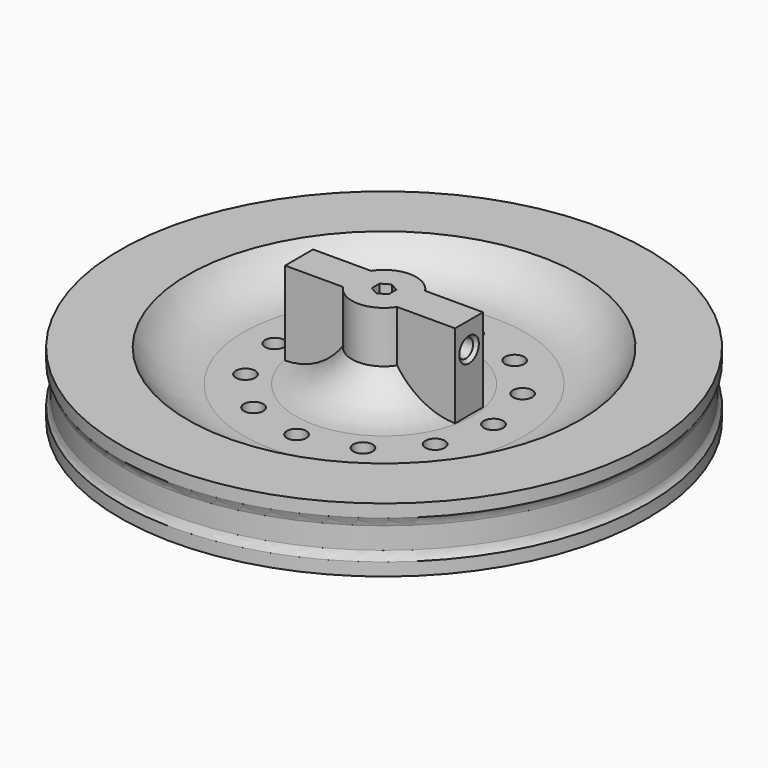
from build123d import *

# Parameters (mm, degrees)
F5_DEPTH  = 8
F6_DEPTH  = 9
F7_R      = 1.4
F8_DEPTH  = 54.201
F10_DEPTH = 18.001
F12_DEPTH = 26.4
F14_DEPTH = 18.001
F16_DEPTH = 5
F17_SIZE  = 0.5
F18_R     = 1.5
F19_DEPTH = 18.0010001


# Not quite as in the source:
# - a fillet or chamfer that OpenCascade refuses, or shapes differently, is made with other operations: its cross-section is extruded or revolved along the edge and cut away or added


with BuildPart() as f1:
    # F0 (on Front) → F1 (revolve)
    with BuildSketch(Plane.XZ):
        Polygon((0, 10), (0, 0), (41, 0), (41, 2), (40.5, 2), (40.5, 8), (41, 8), (41, 10), (30.5, 10), (30.5, 5), (5, 5), (5, 10), align=None)
    revolve(axis=Axis((0, 0, 5), (0, 0, -1)))

    # F2: fillet of radius 10 on 1 edges, made by hand

    # F2_s1 → F2_t2 (revolve)
    with BuildSketch(Plane.XZ):
        with BuildLine():
            ThreePointArc((13.6602540378, 5), (8.6602540378, 6.3397459622), (5, 10))
            Line((5, 10), (5, 5))
            Line((5, 5), (13.6602540378, 5))
        make_face()
    revolve(axis=Axis((0, 0, 5), (0, 0, -1)))

    # F3: fillet of radius 10 on 1 edges, made by hand

    # F3_s1 → F3_t2 (revolve)
    with BuildSketch(Plane.XZ):
        with BuildLine():
            ThreePointArc((30.5, 10), (26.8397459622, 6.3397459622), (21.8397459622, 5))
            Line((21.8397459622, 5), (30.5, 5))
            Line((30.5, 5), (30.5, 10))
        make_face()
    revolve(axis=Axis((0, 0, 5), (0, 0, -1)))

    # F4 (on face) → F5 (join)
    with BuildSketch(Plane.XY.offset(10)):
        with BuildLine():
            Line((-4.2, 2.7129319933), (-4.2, -2.7129319933))
            ThreePointArc((-4.2, -2.7129319933), (5, 0), (-4.2, 2.7129319933))
        make_face()
        Polygon((1.3, -0.7505553499), (0, -1.5011106999), (-1.3, -0.7505553499), (-1.3, 0.7505553499), (0, 1.5011106999), (1.3, 0.7505553499), align=None, mode=Mode.SUBTRACT)
    extrude(amount=F5_DEPTH)

    # F6 (add): a face of the model
    f6_faces = [f1.faces().sort_by_distance(p)[0] for p in [
        (-4.2, 0, 14),
    ]]
    extrude(f6_faces, amount=F6_DEPTH)

    # F7 (on face) → F8 (cut, through all)
    with BuildSketch(Plane(origin=(-13.2, 0, 0), x_dir=(0, -1, 0), z_dir=(-1, 0, 0))):
        with Locations((0, 14)):
            Circle(F7_R)
    extrude(amount=-F8_DEPTH, mode=Mode.SUBTRACT)

    # F9 (on face) → F10 (cut, through all)
    with BuildSketch(Plane.XY.offset(18)):
        Polygon((0, -1.5011106999), (1.3, -0.7505553499), (1.3, 0.7505553499), (0, 1.5011106999), (-1.3, 0.7505553499), (-1.3, -0.7505553499), align=None)
    extrude(amount=-F10_DEPTH, mode=Mode.SUBTRACT)

    # F11: fillet of radius 2 on 2 edges, made by hand

    # F11_s1 → F11_t2 (revolve)
    with BuildSketch(Plane.XZ):
        with BuildLine():
            ThreePointArc((40.5, 3.3228756555), (40.6291713066, 2.6157688743), (41, 2))
            Line((41, 2), (40.5, 2))
            Line((40.5, 2), (40.5, 3.3228756555))
        make_face()
    revolve(axis=Axis((0, 0, 2), (0, 0, -1)))

    # F11_s3 → F11_t4 (revolve)
    with BuildSketch(Plane.XZ):
        with BuildLine():
            ThreePointArc((41, 8), (40.6291713066, 7.3842311257), (40.5, 6.6771243445))
            Line((40.5, 6.6771243445), (40.5, 8))
            Line((40.5, 8), (41, 8))
        make_face()
    revolve(axis=Axis((0, 0, 8), (0, 0, -1)))

    # F12 (add): a face of the model
    f12_faces = [f1.faces().sort_by_distance(p)[0] for p in [
        (-13.2, 2.6162676255, 14),
    ]]
    extrude(f12_faces, amount=-F12_DEPTH)

    # F13 (on face) → F14 (cut, through all)
    with BuildSketch(Plane(origin=(0, 0, 0), x_dir=(1, 0, 0), z_dir=(0, 0, -1))):
        Polygon((0, -1.5011106999), (1.3, -0.7505553499), (1.3, 0.7505553499), (0, 1.5011106999), (-1.3, 0.7505553499), (-1.3, -0.7505553499), align=None)
    extrude(amount=-F14_DEPTH, mode=Mode.SUBTRACT)

    # F15 (on face) → F16 (join, through all)
    with BuildSketch(Plane.XY.offset(10)):
        with BuildLine():
            Line((13.2, -2.7129319933), (13.2, 2.7129319933))
            Line((13.2, 2.7129319933), (4.2, 2.7129319933))
            ThreePointArc((4.2, 2.7129319933), (0, 5), (-4.2, 2.7129319933))
            Line((-4.2, 2.7129319933), (-13.2, 2.7129319933))
            Line((-13.2, 2.7129319933), (-13.2, -2.7129319933))
            Line((-13.2, -2.7129319933), (-4.2, -2.7129319933))
            ThreePointArc((-4.2, -2.7129319933), (0, -5), (4.2, -2.7129319933))
            Line((4.2, -2.7129319933), (13.2, -2.7129319933))
        make_face()
    extrude(amount=-F16_DEPTH)

    # F17
    f17_edges = [f1.edges().sort_by_distance(p)[0] for p in [
        (-13.2, 1.4, 14),
        (13.2, 1.4, 14),
    ]]
    chamfer(f17_edges, length=F17_SIZE)

    # F18 (on face) → F19 (cut, through all)
    with BuildSketch(Plane(origin=(0, 0, 0), x_dir=(1, 0, 0), z_dir=(0, 0, -1))):
        with Locations((0, 17)):
            Circle(F18_R)
        with Locations((-8.5, 14.7224318643)):
            Circle(F18_R)
        with Locations((-14.7224318643, 8.5)):
            Circle(F18_R)
        with Locations((-17, 0)):
            Circle(F18_R)
        with Locations((-14.7224318643, -8.5)):
            Circle(F18_R)
        with Locations((-8.5, -14.7224318643)):
            Circle(F18_R)
        with Locations((0, -17)):
            Circle(F18_R)
        with Locations((8.5, -14.7224318643)):
            Circle(F18_R)
        with Locations((14.7224318643, -8.5)):
            Circle(F18_R)
        with Locations((17, 0)):
            Circle(F18_R)
        with Locations((14.7224318643, 8.5)):
            Circle(F18_R)
        with Locations((8.5, 14.7224318643)):
            Circle(F18_R)
    extrude(amount=-F19_DEPTH, mode=Mode.SUBTRACT)


solid = f1.part
